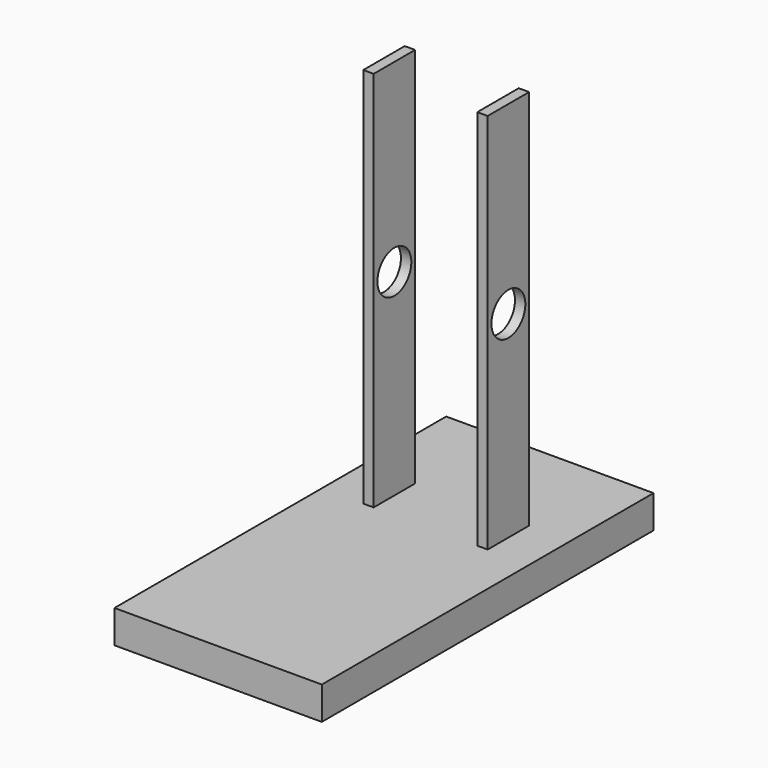
from build123d import *

# Parameters (mm, degrees)
F0_W     = 20
F0_H     = 40
F0_W_2   = 1
F0_H_2   = 5
F1_DEPTH = 3.175
F2_DEPTH = 40
F4_D     = 4.0894


# Not quite as in the source:
# - a length typed as a fraction of an inch, garbled in the dataset ("3 / 203.2 mm" for 3/8 in), is restored


with BuildPart() as f1:
    # F0 (on Top) → F1 (new body)
    with BuildSketch(Plane.XY):
        Rectangle(F0_W, F0_H)
        with Locations((-5.5, 7.5)):
            Rectangle(F0_W_2, F0_H_2, mode=Mode.SUBTRACT)
        with Locations((5.5, 7.5)):
            Rectangle(F0_W_2, F0_H_2, mode=Mode.SUBTRACT)
    extrude(amount=F1_DEPTH)

    # F0 (on Top) → F2 (join)
    with BuildSketch(Plane.XY):
        with Locations((-5.5, 7.5)):
            Rectangle(F0_W_2, F0_H_2)
        with Locations((5.5, 7.5)):
            Rectangle(F0_W_2, F0_H_2)
    extrude(amount=F2_DEPTH)

    # F4 (through all)
    with Locations(Plane.YZ.offset(6)):
        with Locations((7.5, 22.175)):
            Hole(F4_D / 2)


solid = f1.part
